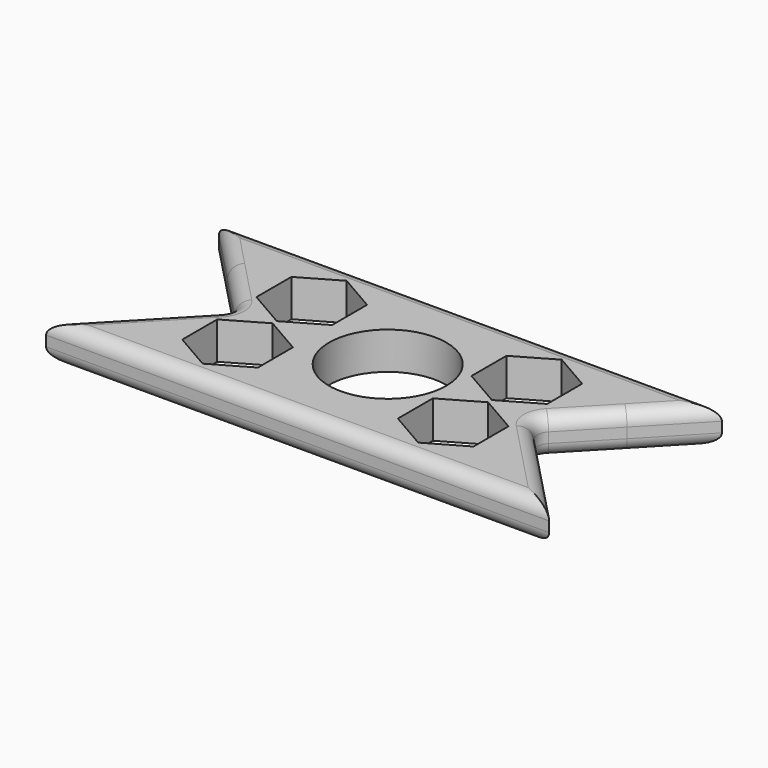
from build123d import *

# Parameters (mm, degrees)
F0_R      = 11
F1_DEPTH  = 7
F2_F1_R   = 2.54
F2_F2_R   = 2.54
F7_DEPTH  = 7.001
F8_DEPTH  = 7.001
F9_DEPTH  = 7.001
F10_DEPTH = 7.001


with BuildPart() as f1:
    # F0 (on Top) → F1 (new body)
    with BuildSketch(Plane.XY):
        Polygon((-46.5175881982, -16.4707175266), (1.3742837651, -16.4707175266), (47.8816837651, -16.4707175266), (38.1750466591, -6.3388262363), (28.4684095532, 3.7930650539), (38.1750466591, 13.9249563442), (47.8816837651, 24.0568476345), (1.3742837651, 24.0568476345), (-46.5175881982, 24.0568476345), (-36.8075984385, 13.9249563442), (-27.0976086789, 3.7930650539), (-36.8075984385, -6.3388262363), align=None)
        with Locations((1.3742837651, 3.7930650539)):
            Circle(F0_R, mode=Mode.SUBTRACT)
    extrude(amount=F1_DEPTH)

    # F2: fillet of radius 2.54 on 10 edges, made by hand

    # F2_f1
    f2_f1_edges = [f1.edges().sort_by_distance(p)[0] for p in [
        (28.4684095532, 3.7930650539, 3.5),
        (-27.0976086789, 3.7930650539, 3.5),
    ]]
    fillet(f2_f1_edges, radius=F2_F1_R)

    # F2_f2
    f2_f2_edges = [f1.edges().sort_by_distance(p)[0] for p in [
        (0.6820477835, -16.4707175266, 7),
        (0.6820477835, 24.0568476345, 7),
        (0.6820477835, 24.0568476345, 0),
        (0.6820477835, -16.4707175266, 0),
        (39.0167452033, -7.2174001498, 7),
        (-37.649739308, 14.8036884491, 7),
        (-37.649739308, -7.2175583413, 0),
        (39.0167452033, 14.8035302576, 0),
        (29.4459362755, 3.7930650539, 0),
        (-28.0757168957, 3.7930650539, 0),
        (-28.0757168957, 3.7930650539, 7),
        (29.4459362755, 3.7930650539, 7),
    ]]
    fillet(f2_f2_edges, radius=F2_F2_R)

    # F3 (on face) → F7 (cut, through all)
    with BuildSketch(Plane.XY.offset(7)):
        Polygon((-12.7487120452, 8.4079941735), (-12.7487120452, 16.6059941735), (-19.8483883054, 20.7049941735), (-26.9480645657, 16.6059941735), (-26.9480645657, 8.4079941735), (-19.8483883054, 4.3089941735), align=None)
    extrude(amount=-F7_DEPTH, mode=Mode.SUBTRACT)

    # F4 (on face) → F8 (cut, through all)
    with BuildSketch(Plane.XY.offset(7)):
        Polygon((-12.8069793108, -8.9152967557), (-12.8069793108, -0.7172967557), (-19.906655571, 3.3817032443), (-27.0063318312, -0.7172967557), (-27.0063318312, -8.9152967557), (-19.906655571, -13.0142967557), align=None)
    extrude(amount=-F8_DEPTH, mode=Mode.SUBTRACT)

    # F6 (on face) → F9 (cut, through all)
    with BuildSketch(Plane.XY.offset(7)):
        Polygon((27.5151642737, -8.7466302544), (27.5151642737, -0.5486302544), (20.4154880135, 3.5503697456), (13.3158117533, -0.5486302544), (13.3158117533, -8.7466302544), (20.4154880135, -12.8456302544), align=None)
    extrude(amount=-F9_DEPTH, mode=Mode.SUBTRACT)

    # F5 (on face) → F10 (cut, through all)
    with BuildSketch(Plane.XY.offset(7)):
        Polygon((27.5004574447, 8.5391272614), (27.5004574447, 16.7371272614), (20.4007811844, 20.8361272614), (13.3011049242, 16.7371272614), (13.3011049242, 8.5391272614), (20.4007811844, 4.4401272614), align=None)
    extrude(amount=-F10_DEPTH, mode=Mode.SUBTRACT)


solid = f1.part
